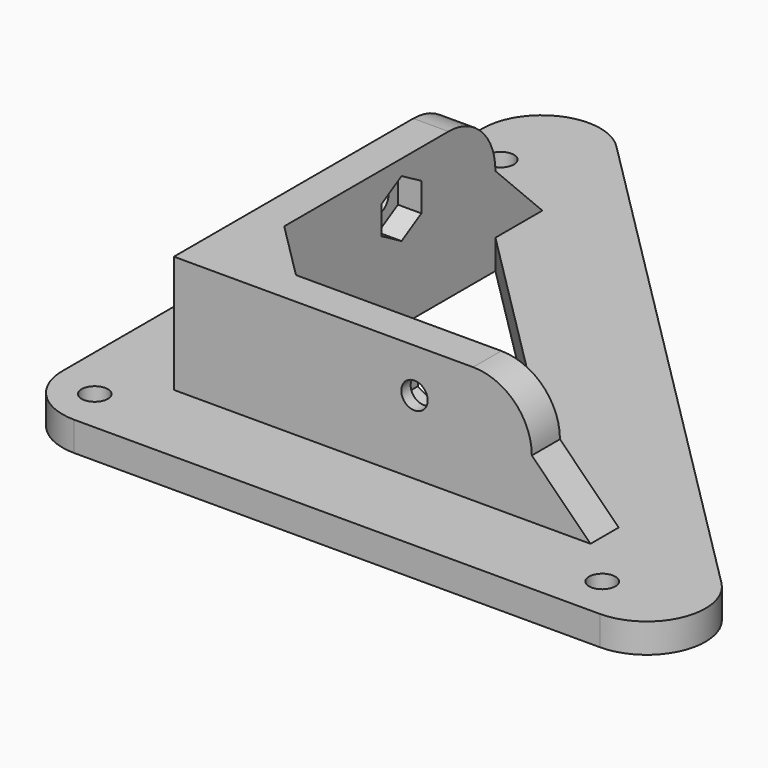
from build123d import *

# Parameters (mm, degrees)
F0_R      = 2.25
F1_DEPTH  = 5
F3_DEPTH  = 20
F4_R      = 10
F5_R      = 2.25
F6_DEPTH  = 25
F7_R      = 2.25
F8_DEPTH  = 25
F9_SIZE   = 9.99999
F11_DEPTH = 4
F13_DEPTH = 4


# Not quite as in the source:
# - a fillet or chamfer is up to 0.001 mm smaller than in the source, because OpenCascade refuses the exact size


with BuildPart() as f1:
    # F0 (on Top) → F1 (new body)
    with BuildSketch(Plane.XY):
        Polygon((123.7436867076, 0), (0, 123.7436867076), (0, 103.7436867076), (0, 0), (103.7436867076, 0), align=None)
        with Locations((7.5, 7.5)):
            Circle(F0_R, mode=Mode.SUBTRACT)
        Polygon((21, 21), (21, 76), (76, 21), align=None, mode=Mode.SUBTRACT)
        with Locations((94, 7.5)):
            Circle(F0_R, mode=Mode.SUBTRACT)
        with Locations((7.5, 94)):
            Circle(F0_R, mode=Mode.SUBTRACT)
    extrude(amount=F1_DEPTH)

    # F2 (on face) → F3 (join)
    with BuildSketch(Plane.XY.offset(5)):
        Polygon((76, 15), (76, 21), (21, 21), (21, 76), (15, 76), (15, 15), align=None)
    extrude(amount=F3_DEPTH)

    # F4
    f4_edges = [f1.edges().sort_by_distance(p)[0] for p in [
        (0, 123.743687, 2.5),
        (123.743687, 0, 2.5),
        (76, 18, 25),
        (18, 76, 25),
        (0, 0, 2.5),
    ]]
    fillet(f4_edges, radius=F4_R)

    # F5 (on face) → F6 (cut)
    with BuildSketch(Plane.YZ.offset(21)):
        with Locations((56, 17.5)):
            Circle(F5_R)
    extrude(amount=-F6_DEPTH, mode=Mode.SUBTRACT)

    # F7 (on face) → F8 (cut)
    with BuildSketch(Plane(origin=(0, 21, 0), x_dir=(-1, 0, 0), z_dir=(0, 1, 0))):
        with Locations((-56, 17.5)):
            Circle(F7_R)
    extrude(amount=-F8_DEPTH, mode=Mode.SUBTRACT)

    # F9 (size 10 in the source; OpenCascade refuses exactly that, so slightly less here)
    f9_edges = [f1.edges().sort_by_distance(p)[0] for p in [
        (18, 76, 5),
        (76, 18, 5),
        (21, 21, 12.5),
    ]]
    chamfer(f9_edges, length=F9_SIZE)

    # F10 (on face) → F11 (cut)
    with BuildSketch(Plane(origin=(0, 21, 0), x_dir=(-1, 0, 0), z_dir=(0, 1, 0))):
        Polygon((-51.775, 15.0606951127), (-51.775, 19.9393048873), (-56, 22.3786097747), (-60.225, 19.9393048873), (-60.225, 15.0606951127), (-56, 12.6213902253), align=None)
    extrude(amount=-F11_DEPTH, mode=Mode.SUBTRACT)

    # F12 (on face) → F13 (cut)
    with BuildSketch(Plane.YZ.offset(21)):
        Polygon((60.225, 15.0606951127), (60.225, 19.9393048873), (56, 22.3786097747), (51.775, 19.9393048873), (51.775, 15.0606951127), (56, 12.6213902253), align=None)
    extrude(amount=-F13_DEPTH, mode=Mode.SUBTRACT)


solid = f1.part
